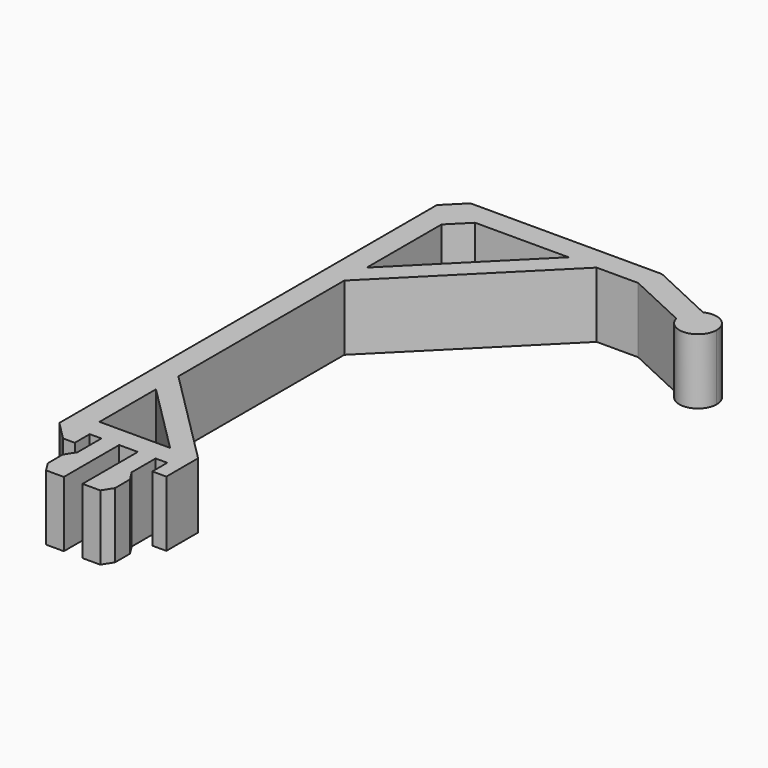
from build123d import *

# Parameters (mm, degrees)
F1_DEPTH = 7
F2_SIZE  = 2


with BuildPart() as f1:
    # F0 (on Top) → F1 (new body)
    with BuildSketch(Plane.XY):
        Polygon((-1, -7.4), (-1, 0), (-2.9, 0), (-2.9, -3.2000038773), (-2.9, -7.4), align=None)
        with BuildLine():
            Line((-2.9, 0), (-1, 0))
            Line((-1, 0), (1, 0))
            Line((1, 0), (2.9, 0))
            Line((2.9, 0), (4.15, 0))
            Line((4.15, 0), (4.15, -2))
            Line((4.15, -2), (5.65, -2))
            Line((5.65, -2), (5.65, 2.25))
            Line((5.65, 2.25), (-4.9, 12.8))
            Line((-4.9, 12.8), (-4.9, 35))
            Line((-4.9, 35), (-4.9, 38))
            Line((-4.9, 38), (-4.9, 50))
            Line((-4.9, 50), (7.1, 50))
            Line((7.1, 50), (10.1, 50))
            Line((10.1, 50), (14.5457633434, 50))
            Line((14.5457633434, 50), (21.060983901, 46.9619027594))
            ThreePointArc((21.060983901, 46.9619027594), (21.1916137331, 48.280211467), (22.1175295553, 49.227672227))
            Line((22.1175295553, 49.227672227), (15.1, 52.5))
            Line((15.1, 52.5), (-7.4, 52.5))
            Line((-7.4, 52.5), (-7.4, -2))
            Line((-7.4, -2), (-4.15, -2))
            Line((-4.15, -2), (-4.15, 0))
            Line((-4.15, 0), (-2.9, 0))
        make_face()
        Polygon((-4.9, 9.8), (2.65, 2.25), (-4.9, 2.25), align=None, mode=Mode.SUBTRACT)
        Polygon((2.9, 0), (1, 0), (1, -7.4), (2.9, -7.4), (2.9, -3.2000038773), align=None)
        Polygon((-2.9, -7.4), (-2.9, -3.2000038773), (-3.6, -4.3000019386), (-3.6, -6.3000019386), align=None)
        Polygon((3.6, -4.3000019386), (2.9, -3.2000038773), (2.9, -7.4), (3.6, -6.3000019386), align=None)
        with BuildLine():
            ThreePointArc((25.0042293071, 47.4349749436), (24.0593597485, 49.1340040051), (22.1175295553, 49.227672227))
            Line((22.1175295553, 49.227672227), (23.5325021343, 48.5678596774))
            Line((23.5325021343, 48.5678596774), (22.47595648, 46.3020902098))
            Line((22.47595648, 46.3020902098), (21.060983901, 46.9619027594))
            ThreePointArc((21.060983901, 46.9619027594), (23.2424615338, 45.4492142817), (25.0042293071, 47.4349749436))
        make_face()
        with BuildLine():
            Line((23.5325021343, 48.5678596774), (22.1175295553, 49.227672227))
            ThreePointArc((22.1175295553, 49.227672227), (21.1916137331, 48.280211467), (21.060983901, 46.9619027594))
            Line((21.060983901, 46.9619027594), (22.47595648, 46.3020902098))
            Line((22.47595648, 46.3020902098), (23.5325021343, 48.5678596774))
        make_face()
        Polygon((-4.9, 38), (-4.9, 35), (10.1, 50), (7.1, 50), align=None)
    extrude(amount=F1_DEPTH)

    # F2
    f2_edges = [f1.edges().sort_by_distance(p)[0] for p in [
        (-4.9, 50, 3.5),
        (-7.4, 52.5, 3.5),
        (-7.4, -2, 3.5),
    ]]
    chamfer(f2_edges, length=F2_SIZE)


solid = f1.part
